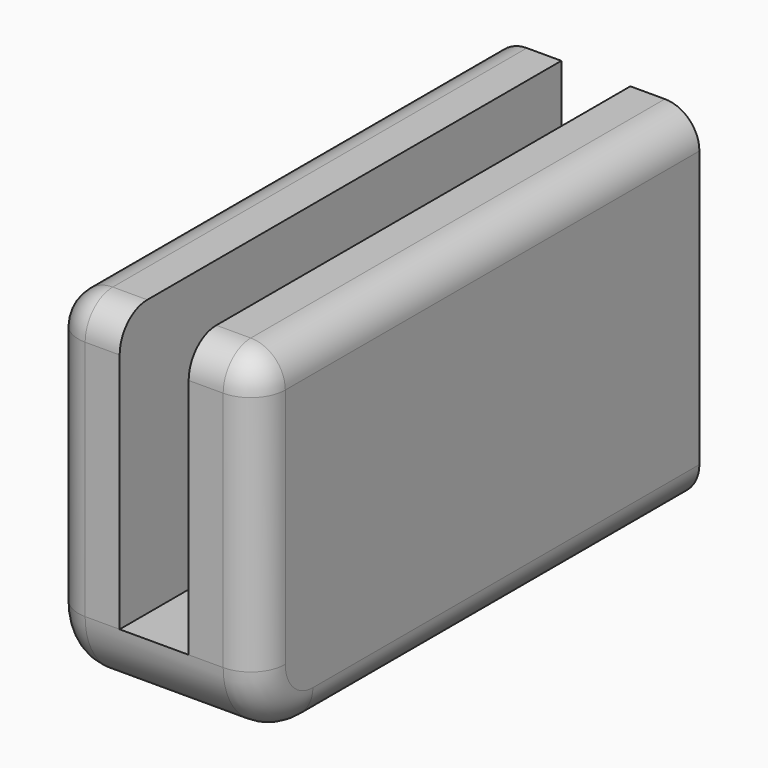
from build123d import *

# Parameters (mm, degrees)
F1_DEPTH = 8
F2_R     = 0.99999
F3_R     = 0.5


# Not quite as in the source:
# - a fillet or chamfer is up to 0.001 mm smaller than in the source, because OpenCascade refuses the exact size


with BuildPart() as f1:
    # F0 (on Front) → F1 (new body)
    with BuildSketch(Plane.XZ):
        Polygon((1.5, -2.5), (1.5, 2.5), (0.5, 2.5), (0.5, -1.5), (-0.5, -1.5), (-0.5, 2.5), (-1.5, 2.5), (-1.5, -2.5), align=None)
    extrude(amount=F1_DEPTH)

    # F2 (radius 1 in the source; OpenCascade refuses exactly that, so slightly less here)
    f2_edges = [f1.edges().sort_by_distance(p)[0] for p in [
        (0, -8, -2.5),
    ]]
    fillet(f2_edges, radius=F2_R)

    # F3
    f3_edges = [f1.edges().sort_by_distance(p)[0] for p in [
        (-1.5, -3.500005, -2.5),
        (1.5, -3.500005, -2.5),
        (1.5, -4, 2.5),
        (-1.5, -4, 2.5),
        (-1, -8, 2.5),
        (1, -8, 2.5),
    ]]
    fillet(f3_edges, radius=F3_R)


solid = f1.part
